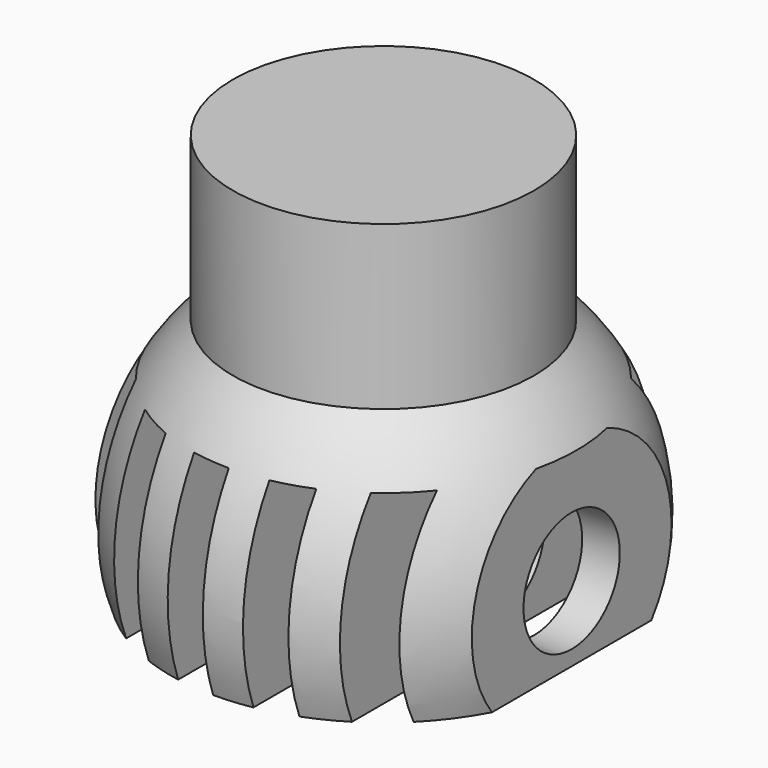
from build123d import *

# Parameters (mm, degrees)
F0_W            = 10
F0_H            = 7
F6_DEPTH        = 30.001
F6_COPIES_COUNT = 2
F6_COPIES_PITCH = 25
F9_R            = 4
F10_DEPTH       = 27.8451708576


# Not quite as in the source:
# - a pattern or mirror of a feature is missing from the dataset's text; its kind, count and spacing are read off the source's solid


with BuildPart() as f1:
    # F0 (on Front) → F1 (revolve)
    with BuildSketch(Plane.XZ):
        with BuildLine():
            Line((0, -5), (0, 15))
            ThreePointArc((0, 15), (-5.3523313466, 14.0125853844), (-10, 11.1803398875))
            ThreePointArc((-10, 11.1803398875), (-14.5313980001, 3.7200096993), (-14.1421356237, -5))
            Line((-14.1421356237, -5), (0, -5))
        make_face()
        with BuildLine():
            ThreePointArc((-10, 11.1803398875), (-5.3523313466, 14.0125853844), (0, 15))
            Line((0, 15), (-10, 15))
            Line((-10, 15), (-10, 11.1803398875))
        make_face()
        with Locations((-5, 18.5)):
            Rectangle(F0_W, F0_H)
    revolve(axis=Axis((0, 0, 18.5), (0, 0, 1)))

    # F5 (on line) → F6 (cut, through all)
    with BuildSketch(Plane(origin=(0, 15, 0), x_dir=(-1, 0, 0), z_dir=(0, 1, 0))):
        with BuildLine():
            Line((-7.5, -12.9903810568), (-7.5, 7.7477270849))
            Line((-7.5, 7.7477270849), (-10, 7.7477270849))
            Line((-10, 7.7477270849), (-10, -11.1803398875))
            ThreePointArc((-10, -11.1803398875), (-8.7966790472, -12.1498328277), (-7.5, -12.9903810568))
        make_face()
        with BuildLine():
            Line((-2.5, 7.7477270849), (-5, 7.7477270849))
            Line((-5, 7.7477270849), (-5, -14.1421356237))
            ThreePointArc((-5, -14.1421356237), (-3.7639735232, -14.5200724281), (-2.5, -14.7901994577))
            Line((-2.5, -14.7901994577), (-2.5, 7.7477270849))
        make_face()
        with BuildLine():
            Line((2.5, 7.7477270849), (0, 7.7477270849))
            Line((0, 7.7477270849), (0, -15))
            ThreePointArc((0, -15), (1.2543939042, -14.9474578418), (2.5, -14.7901994577))
            Line((2.5, -14.7901994577), (2.5, 7.7477270849))
        make_face()
        with BuildLine():
            Line((7.5, 7.7477270849), (5, 7.7477270849))
            Line((5, 7.7477270849), (5, -14.1421356237))
            ThreePointArc((5, -14.1421356237), (6.2764746989, -13.623724357), (7.5, -12.9903810568))
            Line((7.5, -12.9903810568), (7.5, 7.7477270849))
        make_face()
        with BuildLine():
            Line((12.5, 7.7477270849), (10, 7.7477270849))
            Line((10, 7.7477270849), (10, -11.1803398875))
            ThreePointArc((10, -11.1803398875), (11.3423436492, -9.815866775), (12.5, -8.2915619759))
            Line((12.5, -8.2915619759), (12.5, 7.7477270849))
        make_face()
    f6 = extrude(amount=-F6_DEPTH, mode=Mode.SUBTRACT)

    # F6_copies: F6 ×2
    with Locations(*[(i * F6_COPIES_PITCH, 0, 0) for i in range(1, F6_COPIES_COUNT)]):
        add(f6, mode=Mode.SUBTRACT)

    # F9 (on line) → F10 (cut, through all)
    with BuildSketch(Plane(origin=(-15, 0, 0), x_dir=(0, -1, 0), z_dir=(-1, 0, 0))):
        Circle(F9_R)
    extrude(amount=-F10_DEPTH, mode=Mode.SUBTRACT)


solid = f1.part
